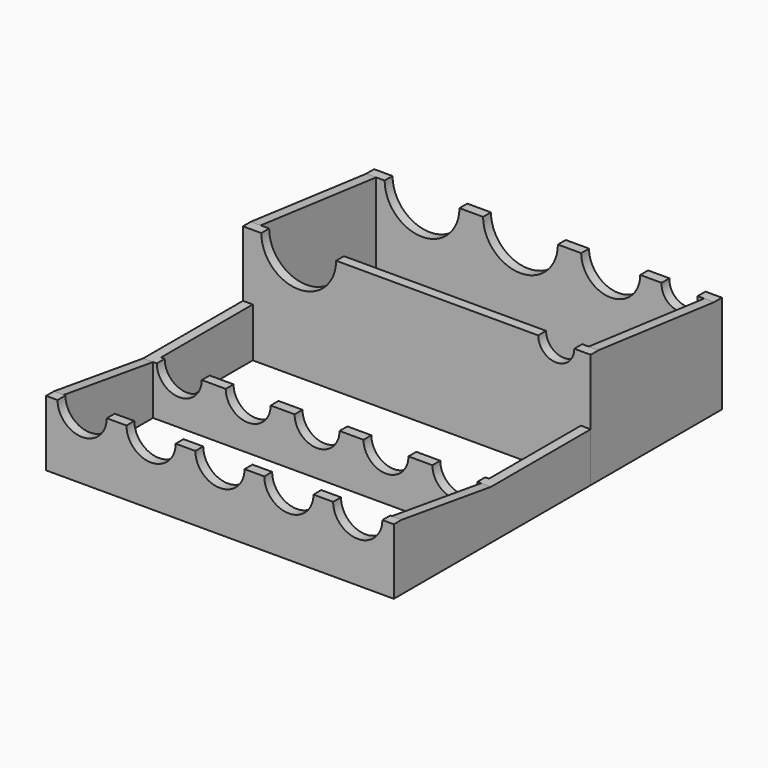
from build123d import *

# Parameters (mm, degrees)
F0_W      = 106
F0_H      = 40
F1_DEPTH  = 20
F2_W      = 100
F2_H      = 34
F3_DEPTH  = 20
F6_DEPTH  = 3
F7_W      = 106
F7_H      = 5
F8_DEPTH  = 3
F10_DEPTH = 3
F12_W     = 35
F12_H     = 15
F13_DEPTH = 3
F11_W     = 35
F11_H     = 15
F14_DEPTH = 3
F15_W     = 100
F15_H     = 44
F16_DEPTH = 35
F18_DEPTH = 3
F20_DEPTH = 3
F22_DEPTH = 3
F23_W     = 106
F23_H     = 5
F24_DEPTH = 3
F26_DEPTH = 3
F28_DEPTH = 3
F30_DEPTH = 3


# Not quite as in the source:
# - a feature names something its author has since deleted; it is built from what else it names


with BuildPart() as f1:
    # F0 (on Top) → F1 (new body)
    with BuildSketch(Plane.XY):
        with Locations((0.6567015983, -32.3096490646)):
            Rectangle(F0_W, F0_H)
    extrude(amount=F1_DEPTH)

    # F2 (on face) → F3 (cut)
    with BuildSketch(Plane.XY.offset(20)):
        with Locations((0.6567015983, -32.3096490646)):
            Rectangle(F2_W, F2_H)
    extrude(amount=-F3_DEPTH, mode=Mode.SUBTRACT)

    # F5 (on face) + F4 (on face) → F6 (cut)
    with BuildSketch(Plane.XZ.offset(52.3096490646)):
        with BuildLine():
            ThreePointArc((-33.8432984017, 20), (-41.3432984017, 27.5), (-48.8432984017, 20))
            Line((-48.8432984017, 20), (-33.8432984017, 20))
        make_face()
    with BuildSketch(Plane.XZ.offset(52.3096490646)):
        with BuildLine():
            ThreePointArc((-48.8432984017, 20), (-41.3432984017, 12.5), (-33.8432984017, 20))
            Line((-33.8432984017, 20), (-48.8432984017, 20))
        make_face()
        with BuildLine():
            Line((-12.8432984017, 20), (-27.8432984017, 20))
            ThreePointArc((-27.8432984017, 20), (-20.3432984017, 12.5), (-12.8432984017, 20))
        make_face()
        with BuildLine():
            Line((8.1567015983, 20), (-6.8432984017, 20))
            ThreePointArc((-6.8432984017, 20), (0.6567015983, 12.5), (8.1567015983, 20))
        make_face()
        with BuildLine():
            Line((29.1567015983, 20), (14.1567015983, 20))
            ThreePointArc((14.1567015983, 20), (21.6567015983, 12.5), (29.1567015983, 20))
        make_face()
        with BuildLine():
            ThreePointArc((35.1567015983, 20), (42.6567015983, 12.5), (50.1567015983, 20))
            Line((50.1567015983, 20), (35.1567015983, 20))
        make_face()
    extrude(amount=-F6_DEPTH, mode=Mode.SUBTRACT)

    # F7 (on face) → F8 (cut)
    with BuildSketch(Plane(origin=(0, -12.3096490646, 0), x_dir=(-1, 0, 0), z_dir=(0, 1, 0))):
        with Locations((-0.6567015983, 17.5)):
            Rectangle(F7_W, F7_H)
    extrude(amount=-F8_DEPTH, mode=Mode.SUBTRACT)

    # F9 (on face) → F10 (cut)
    with BuildSketch(Plane(origin=(0, -12.3096490646, 0), x_dir=(-1, 0, 0), z_dir=(0, 1, 0))):
        with BuildLine():
            Line((34.4932984017, 15), (48.1932984017, 15))
            ThreePointArc((48.1932984017, 15), (41.3432984017, 21.85), (34.4932984017, 15))
        make_face()
        with BuildLine():
            ThreePointArc((34.4932984017, 15), (41.3432984017, 8.15), (48.1932984017, 15))
            Line((48.1932984017, 15), (34.4932984017, 15))
        make_face()
        with BuildLine():
            Line((13.4932984017, 15), (27.1932984017, 15))
            ThreePointArc((27.1932984017, 15), (20.3432984017, 21.85), (13.4932984017, 15))
        make_face()
        with BuildLine():
            ThreePointArc((13.4932984017, 15), (20.3432984017, 8.15), (27.1932984017, 15))
            Line((27.1932984017, 15), (13.4932984017, 15))
        make_face()
        with BuildLine():
            Line((-7.5067015983, 15), (6.1932984017, 15))
            ThreePointArc((6.1932984017, 15), (-0.6567015983, 21.85), (-7.5067015983, 15))
        make_face()
        with BuildLine():
            ThreePointArc((-7.5067015983, 15), (-0.6567015983, 8.15), (6.1932984017, 15))
            Line((6.1932984017, 15), (-7.5067015983, 15))
        make_face()
        with BuildLine():
            Line((-35.8067015983, 15), (-49.5067015983, 15))
            ThreePointArc((-49.5067015983, 15), (-42.6567015983, 8.15), (-35.8067015983, 15))
        make_face()
        with BuildLine():
            ThreePointArc((-28.5067015983, 15), (-21.6567015983, 8.15), (-14.8067015983, 15))
            Line((-14.8067015983, 15), (-28.5067015983, 15))
        make_face()
    extrude(amount=-F10_DEPTH, mode=Mode.SUBTRACT)

    # F12 (on face) → F13 (join)
    with BuildSketch(Plane(origin=(-52.3432984017, 0, 0), x_dir=(0, -1, 0), z_dir=(-1, 0, 0))):
        with Locations((-5.1903509354, 7.5)):
            Rectangle(F12_W, F12_H)
    extrude(amount=-F13_DEPTH)

    # F11 (on face) → F14 (join)
    with BuildSketch(Plane.YZ.offset(53.6567015983)):
        with Locations((5.1903509354, 7.5)):
            Rectangle(F11_W, F11_H)
    extrude(amount=-F14_DEPTH)

    # F19 (on face) → F20 (cut)
    with BuildSketch(Plane(origin=(50.6567015983, 0, 0), x_dir=(0, -1, 0), z_dir=(-1, 0, 0))):
        Polygon((15.3096490646, 15), (49.3096490646, 20), (15.3096490646, 20), align=None)
    extrude(amount=-F20_DEPTH, mode=Mode.SUBTRACT)

    # F21 (on face) → F22 (cut)
    with BuildSketch(Plane.YZ.offset(-49.3432984017)):
        Polygon((-15.3096490646, 20), (-49.3096490646, 20), (-15.3096490646, 15), align=None)
    extrude(amount=-F22_DEPTH, mode=Mode.SUBTRACT)


with BuildPart() as f16:
    # F15 (on face) → F16 (new body)
    with BuildSketch(Plane(origin=(0, 0, 0), x_dir=(1, 0, 0), z_dir=(0, 0, -1))):
        Polygon((-49.3432984017, -22.6903509354), (-52.3432984017, -22.6903509354), (-52.3432984017, -72.6903509354), (53.6567015983, -72.6903509354), (53.6567015983, -22.6903509354), (50.6567015983, -22.6903509354), align=None)
        with Locations((0.6567015983, -47.6903509354)):
            Rectangle(F15_W, F15_H, mode=Mode.SUBTRACT)
    extrude(amount=-F16_DEPTH)

    # F17 (on face) → F18 (cut)
    with BuildSketch(Plane.XZ.offset(-22.6903509354)):
        with BuildLine():
            ThreePointArc((-46.7432984017, 35), (-35.3432984017, 23.6), (-23.9432984017, 35))
            Line((-23.9432984017, 35), (-46.7432984017, 35))
        make_face()
        with BuildLine():
            Line((48.6567015983, 35), (37.6567015983, 35))
            ThreePointArc((37.6567015983, 35), (43.1567015983, 29.5), (48.6567015983, 35))
        make_face()
    extrude(amount=-F18_DEPTH, mode=Mode.SUBTRACT)

    # F23 (on face) → F24 (cut)
    with BuildSketch(Plane(origin=(0, 72.6903509354, 0), x_dir=(-1, 0, 0), z_dir=(0, 1, 0))):
        with Locations((-0.6567015983, 32.5)):
            Rectangle(F23_W, F23_H)
    extrude(amount=-F24_DEPTH, mode=Mode.SUBTRACT)

    # F25 (on face) → F26 (cut)
    with BuildSketch(Plane.YZ.offset(-49.3432984017)):
        Polygon((69.6903509354, 35), (25.6903509354, 35), (69.6903509354, 30), align=None)
    extrude(amount=-F26_DEPTH, mode=Mode.SUBTRACT)

    # F27 (on face) → F28 (cut)
    with BuildSketch(Plane(origin=(50.6567015983, 0, 0), x_dir=(0, -1, 0), z_dir=(-1, 0, 0))):
        Polygon((-69.6903509354, 30), (-25.6903509354, 35), (-69.6903509354, 35), align=None)
    extrude(amount=-F28_DEPTH, mode=Mode.SUBTRACT)

    # F29 (on face) → F30 (cut)
    with BuildSketch(Plane.XZ.offset(-69.6903509354)):
        with BuildLine():
            ThreePointArc((-46.7432984017, 30), (-35.3432984017, 18.6), (-23.9432984017, 30))
            Line((-23.9432984017, 30), (-46.7432984017, 30))
        make_face()
        with BuildLine():
            Line((6.0567015983, 30), (-16.7432984017, 30))
            ThreePointArc((-16.7432984017, 30), (-5.3432984017, 18.6), (6.0567015983, 30))
        make_face()
        with BuildLine():
            Line((31.1567015983, 30), (13.1567015983, 30))
            ThreePointArc((13.1567015983, 30), (22.1567015983, 21), (31.1567015983, 30))
        make_face()
        with BuildLine():
            ThreePointArc((31.1567015983, 30), (22.1567015983, 39), (13.1567015983, 30))
            Line((13.1567015983, 30), (31.1567015983, 30))
        make_face()
        with BuildLine():
            Line((48.6423386246, 30), (37.6710645721, 30))
            ThreePointArc((37.6710645721, 30), (42.9579601135, 24.1063685331), (48.6567015983, 29.6027766168))
            ThreePointArc((48.6567015983, 29.6027766168), (48.653109682, 29.8015181016), (48.6423386246, 30))
        make_face()
        with BuildLine():
            ThreePointArc((48.6423386246, 30), (43.1567015983, 35.1027766168), (37.6710645721, 30))
            Line((37.6710645721, 30), (48.6423386246, 30))
        make_face()
    extrude(amount=-F30_DEPTH, mode=Mode.SUBTRACT)


solid = Compound([f1.part, f16.part])
